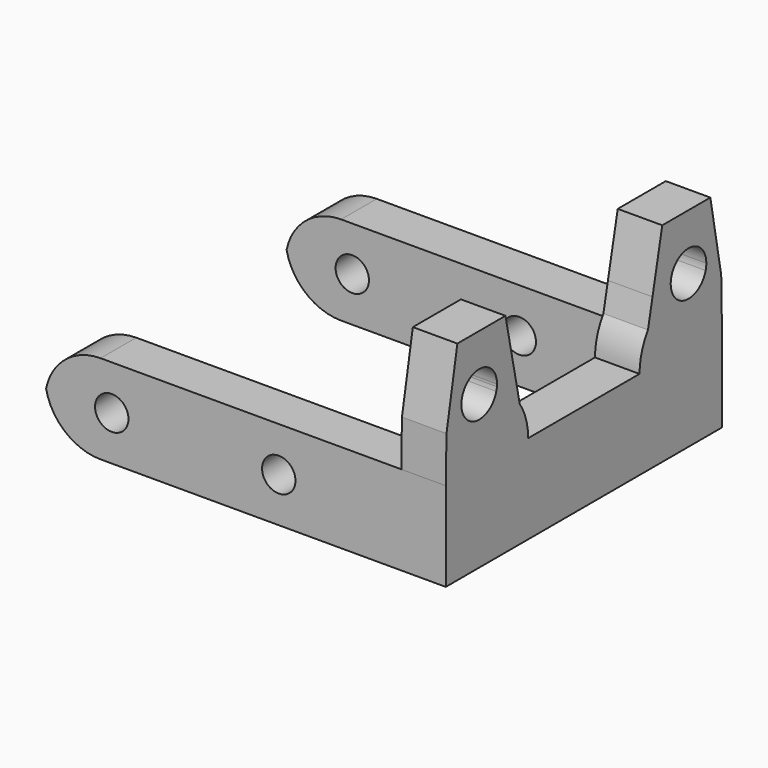
from build123d import *

# Parameters (mm, degrees)
F0_W        = 32
F0_H        = 4
F1_DEPTH    = 8
F3_DEPTH    = 4
F4_DEPTH    = 25
F5_R        = 1.5
F6_DEPTH    = 40
F7_T1_DEPTH = 29
F7_T3_DEPTH = 29


# Not quite as in the source:
# - a fillet or chamfer that OpenCascade refuses, or shapes differently, is made with other operations: its cross-section is extruded or revolved along the edge and cut away or added


with BuildPart() as f1:
    # F0 (on Top) → F1 (new body)
    with BuildSketch(Plane.XY):
        with Locations((-2, 13.5)):
            Rectangle(F0_W, F0_H)
        Polygon((14, 11.5), (14, -11.5), (14, -15.5), (18, -15.5), (18, 0), (18, 15.5), (14, 15.5), align=None)
        with Locations((-2, -13.5)):
            Rectangle(F0_W, F0_H)
    extrude(amount=F1_DEPTH)

    # F2 (on face) → F3 (join, through all)
    with BuildSketch(Plane.YZ.offset(18)):
        with BuildLine():
            Line((-15.4216540828, 12.0949916113), (-15.5, 8))
            Line((-15.5, 8), (-6.25, 8))
            ThreePointArc((-6.25, 8), (-6.4923756022, 9.6147401314), (-7.1981402517, 11.0871625858))
            ThreePointArc((-7.1981402517, 11.0871625858), (-8.3515353126, 12.3244002785), (-9.8263607896, 13.1526315789))
            ThreePointArc((-9.8263607896, 13.1526315789), (-11.75, 11.7), (-13.6736392104, 13.1526315789))
            ThreePointArc((-13.6736392104, 13.1526315789), (-14.5971876184, 12.7056904558), (-15.4216540828, 12.0949916113))
        make_face()
        with BuildLine():
            Line((6.25, 8), (11.75, 8))
            Line((11.75, 8), (15.5, 8))
            Line((15.5, 8), (15.4216540828, 12.0949916113))
            ThreePointArc((15.4216540828, 12.0949916113), (14.5971876184, 12.7056904558), (13.6736392104, 13.1526315789))
            ThreePointArc((13.6736392104, 13.1526315789), (11.75, 11.7), (9.8263607896, 13.1526315789))
            ThreePointArc((9.8263607896, 13.1526315789), (8.3515353126, 12.3244002785), (7.1981402517, 11.0871625858))
            ThreePointArc((7.1981402517, 11.0871625858), (6.4923756022, 9.6147401314), (6.25, 8))
        make_face()
        with BuildLine():
            Line((-14.1999293119, 18.7123082578), (-15.4216540828, 12.0949916113))
            ThreePointArc((-15.4216540828, 12.0949916113), (-14.5971876184, 12.7056904558), (-13.6736392104, 13.1526315789))
            ThreePointArc((-13.6736392104, 13.1526315789), (-12.0263345611, 15.6808178135), (-9.75, 13.7))
            ThreePointArc((-9.75, 13.7), (-9.7525078538, 13.5998744499), (-9.7600251258, 13.5))
            Line((-9.7600251258, 13.5), (-7.7054746686, 13.5))
            Line((-7.7054746686, 13.5), (-8.8014388457, 18.7123082578))
            Line((-8.8014388457, 18.7123082578), (-14.1999293119, 18.7123082578))
        make_face()
        with BuildLine():
            ThreePointArc((-9.8263607896, 13.1526315789), (-8.3515353126, 12.3244002785), (-7.1981402517, 11.0871625858))
            Line((-7.1981402517, 11.0871625858), (-7.7054746686, 13.5))
            Line((-7.7054746686, 13.5), (-9.7600251258, 13.5))
            ThreePointArc((-9.7600251258, 13.5), (-9.7855000622, 13.3248467056), (-9.8263607896, 13.1526315789))
        make_face()
        with BuildLine():
            ThreePointArc((13.6736392104, 13.1526315789), (14.5971876184, 12.7056904558), (15.4216540828, 12.0949916113))
            Line((15.4216540828, 12.0949916113), (14.1999293119, 18.7123082578))
            Line((14.1999293119, 18.7123082578), (8.8014388457, 18.7123082578))
            Line((8.8014388457, 18.7123082578), (7.7054746686, 13.5))
            Line((7.7054746686, 13.5), (9.7600251258, 13.5))
            ThreePointArc((9.7600251258, 13.5), (11.6498744499, 15.6974921462), (13.75, 13.7))
            ThreePointArc((13.75, 13.7), (13.7308178135, 13.4236654389), (13.6736392104, 13.1526315789))
        make_face()
        with BuildLine():
            Line((7.7054746686, 13.5), (7.1981402517, 11.0871625858))
            ThreePointArc((7.1981402517, 11.0871625858), (8.3515353126, 12.3244002785), (9.8263607896, 13.1526315789))
            ThreePointArc((9.8263607896, 13.1526315789), (9.7855000622, 13.3248467056), (9.7600251258, 13.5))
            Line((9.7600251258, 13.5), (7.7054746686, 13.5))
        make_face()
    extrude(amount=-F3_DEPTH)

    # F2 (on face) → F4 (cut)
    with BuildSketch(Plane.YZ.offset(18)):
        with BuildLine():
            ThreePointArc((9.7600251258, 13.5), (9.7855000622, 13.3248467056), (9.8263607896, 13.1526315789))
            ThreePointArc((9.8263607896, 13.1526315789), (10.7726243517, 13.4124612555), (11.75, 13.5))
            Line((11.75, 13.5), (9.7600251258, 13.5))
        make_face()
        with BuildLine():
            ThreePointArc((11.75, 13.5), (10.7726243517, 13.4124612555), (9.8263607896, 13.1526315789))
            ThreePointArc((9.8263607896, 13.1526315789), (11.75, 11.7), (13.6736392104, 13.1526315789))
            ThreePointArc((13.6736392104, 13.1526315789), (12.7273756483, 13.4124612555), (11.75, 13.5))
        make_face()
        with BuildLine():
            ThreePointArc((11.75, 13.5), (12.7273756483, 13.4124612555), (13.6736392104, 13.1526315789))
            ThreePointArc((13.6736392104, 13.1526315789), (13.7308178135, 13.4236654389), (13.75, 13.7))
            ThreePointArc((13.75, 13.7), (11.6498744499, 15.6974921462), (9.7600251258, 13.5))
            Line((9.7600251258, 13.5), (11.75, 13.5))
        make_face()
        with BuildLine():
            ThreePointArc((-11.75, 13.5), (-12.7273756483, 13.4124612555), (-13.6736392104, 13.1526315789))
            ThreePointArc((-13.6736392104, 13.1526315789), (-11.75, 11.7), (-9.8263607896, 13.1526315789))
            ThreePointArc((-9.8263607896, 13.1526315789), (-10.7726243517, 13.4124612555), (-11.75, 13.5))
        make_face()
        with BuildLine():
            ThreePointArc((-11.75, 13.5), (-10.7726243517, 13.4124612555), (-9.8263607896, 13.1526315789))
            ThreePointArc((-9.8263607896, 13.1526315789), (-9.7855000622, 13.3248467056), (-9.7600251258, 13.5))
            Line((-9.7600251258, 13.5), (-11.75, 13.5))
        make_face()
        with BuildLine():
            ThreePointArc((-9.75, 13.7), (-12.0263345611, 15.6808178135), (-13.6736392104, 13.1526315789))
            ThreePointArc((-13.6736392104, 13.1526315789), (-12.7273756483, 13.4124612555), (-11.75, 13.5))
            Line((-11.75, 13.5), (-9.7600251258, 13.5))
            ThreePointArc((-9.7600251258, 13.5), (-9.7525078538, 13.5998744499), (-9.75, 13.7))
        make_face()
    extrude(amount=-F4_DEPTH, mode=Mode.SUBTRACT)

    # F5 (on face) → F6 (cut)
    with BuildSketch(Plane.XZ.offset(15.5)):
        with Locations((-12, 4)):
            Circle(F5_R)
        with Locations((3, 4)):
            Circle(F5_R)
    extrude(amount=-F6_DEPTH, mode=Mode.SUBTRACT)

    # F7: fillet of radius 5 on 4 edges, made by hand

    # F7_s2 → F7_t1 (cut)
    with BuildSketch(Plane.XZ.offset(-1)):
        with BuildLine():
            ThreePointArc((-18, 3), (-16.5355339059, 6.5355339059), (-13, 8))
            Line((-13, 8), (-18, 8))
            Line((-18, 8), (-18, 3))
        make_face()
        with BuildLine():
            ThreePointArc((-13, 0), (-16.5355339059, 1.4644660941), (-18, 5))
            Line((-18, 5), (-18, 0))
            Line((-18, 0), (-13, 0))
        make_face()
    extrude(amount=F7_T1_DEPTH, mode=Mode.SUBTRACT)

    # F7_s4 → F7_t3 (cut)
    with BuildSketch(Plane.XZ.offset(-28)):
        with BuildLine():
            ThreePointArc((-18, 3), (-16.5355339059, 6.5355339059), (-13, 8))
            Line((-13, 8), (-18, 8))
            Line((-18, 8), (-18, 3))
        make_face()
        with BuildLine():
            ThreePointArc((-18, 5), (-16.5355339059, 1.4644660941), (-13, 0))
            Line((-13, 0), (-18, 0))
            Line((-18, 0), (-18, 5))
        make_face()
    extrude(amount=F7_T3_DEPTH, mode=Mode.SUBTRACT)


solid = f1.part
